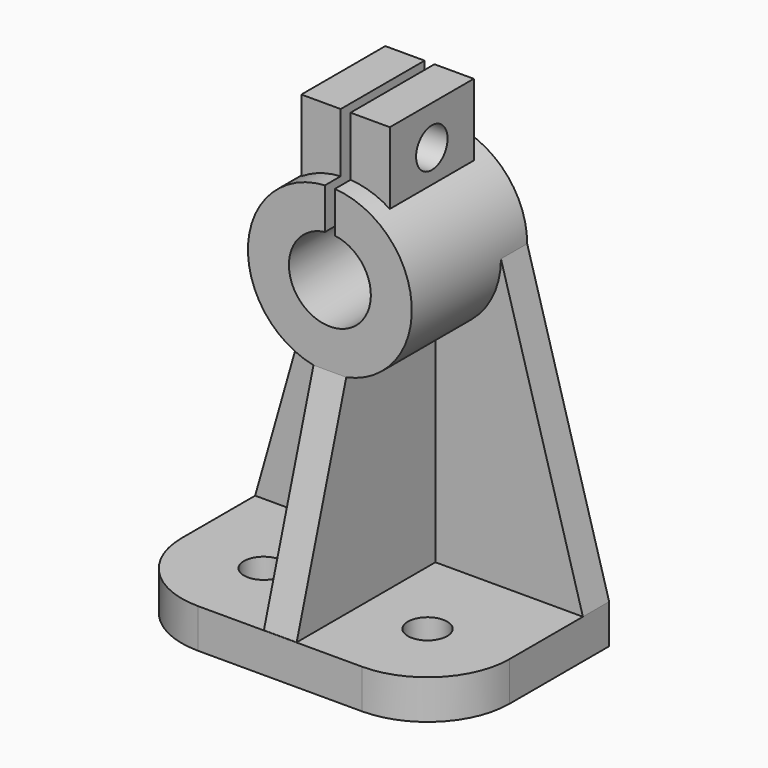
from build123d import *

# Parameters (mm, degrees)
F0_W           = 100
F0_H           = 63
F1_DEPTH       = 12
F2_R           = 25
F3_R           = 6
F4_DEPTH       = 12
F5_R           = 6
F6_DEPTH       = 12
F7_R           = 25
F7_R_2         = 12.5
F8_DEPTH       = 44
F12_DEPTH      = 10
F14_DEPTH      = 10
F16_W          = 27
F16_H          = 32
F17_DEPTH      = 23
F18_W          = 10
F18_H          = 34
F21_DEPTH      = 10
F22_W          = 3
F22_H          = 60
F23_DEPTH      = 25
F23_DEPTH_BACK = 25
F24_R          = 6
F25_DEPTH      = 63.501


# Not quite as in the source:
# - a feature of the source that left no trace in its solid (it failed there, or was rolled back) is left out


with BuildPart() as f1:
    # F0 (on Top) → F1 (new body)
    with BuildSketch(Plane.XY):
        Rectangle(F0_W, F0_H)
    extrude(amount=F1_DEPTH)

    # F2
    f2_edges = [f1.edges().sort_by_distance(p)[0] for p in [
        (-50, -31.5, 6),
        (50, -31.5, 6),
    ]]
    fillet(f2_edges, radius=F2_R)

    # F3 (on face) → F4 (cut, through all)
    with BuildSketch(Plane.XY.offset(12)):
        with Locations((-25, -6.5)):
            Circle(F3_R)
    extrude(amount=-F4_DEPTH, mode=Mode.SUBTRACT)

    # F5 (on face) → F6 (cut, through all)
    with BuildSketch(Plane.XY.offset(12)):
        with Locations((25, -6.5)):
            Circle(F5_R)
    extrude(amount=-F6_DEPTH, mode=Mode.SUBTRACT)



with BuildPart() as f8:
    # F7 (on face) → F8 (new body)
    with BuildSketch(Plane(origin=(0, 31.5, 0), x_dir=(-1, 0, 0), z_dir=(0, 1, 0))):
        with Locations((0, 100)):
            Circle(F7_R)
        with Locations((0, 100)):
            Circle(F7_R_2, mode=Mode.SUBTRACT)
    extrude(amount=-F8_DEPTH)


with BuildPart() as f1_1:
    add(f1.part)

    add(f8.part)  # F12 merges F8
    # F11 (on face) → F12 (join)
    with BuildSketch(Plane(origin=(0, 31.5, 0), x_dir=(-1, 0, 0), z_dir=(0, 1, 0))):
        Polygon((-25, 100), (-50, 12), (-25, 12), align=None)
    extrude(amount=-F12_DEPTH)

    # F13 (on face) → F14 (join)
    with BuildSketch(Plane(origin=(0, 31.5, 0), x_dir=(-1, 0, 0), z_dir=(0, 1, 0))):
        Polygon((25, 100), (25, 12), (50, 12), align=None)
        with BuildLine():
            Line((-25, 12), (25, 12))
            Line((25, 12), (25, 100))
            ThreePointArc((25, 100), (0, 75), (-25, 100))
            Line((-25, 100), (-25, 12))
        make_face()
    extrude(amount=-F14_DEPTH)

    # F16 (on offset) → F17 (join)
    with BuildSketch(Plane.XY.offset(120)):
        with Locations((0, 9.5)):
            Rectangle(F16_W, F16_H)
    extrude(amount=F17_DEPTH)

    # F18 (on face) → F19 (join, up to the next surface of F1)
    with BuildSketch(Plane.XY.offset(12)):
        with Locations((0, 4.5)):
            Rectangle(F18_W, F18_H)
    extrude(until=Until.NEXT)

    # F20 (on face) → F21 (join)
    with BuildSketch(Plane(origin=(-5, 0, 0), x_dir=(0, -1, 0), z_dir=(-1, 0, 0))):
        Polygon((31.4197465777, 12), (12.5, 75.5051025722), (12.5, 12), align=None)
    extrude(amount=-F21_DEPTH)

    # F22 (on offset) → F23 (cut, two sides)
    with BuildSketch(Plane.XY.offset(120)) as f23_sk:
        with Locations((0, 3.3281182433)):
            Rectangle(F22_W, F22_H)
    extrude(amount=-F23_DEPTH, mode=Mode.SUBTRACT)
    extrude(f23_sk.sketch, amount=F23_DEPTH_BACK, mode=Mode.SUBTRACT)

    # F24 (on face) → F25 (cut, through all)
    with BuildSketch(Plane.YZ.offset(13.5)):
        with Locations((9.5, 131)):
            Circle(F24_R)
    extrude(amount=-F25_DEPTH, mode=Mode.SUBTRACT)


solid = f1_1.part
